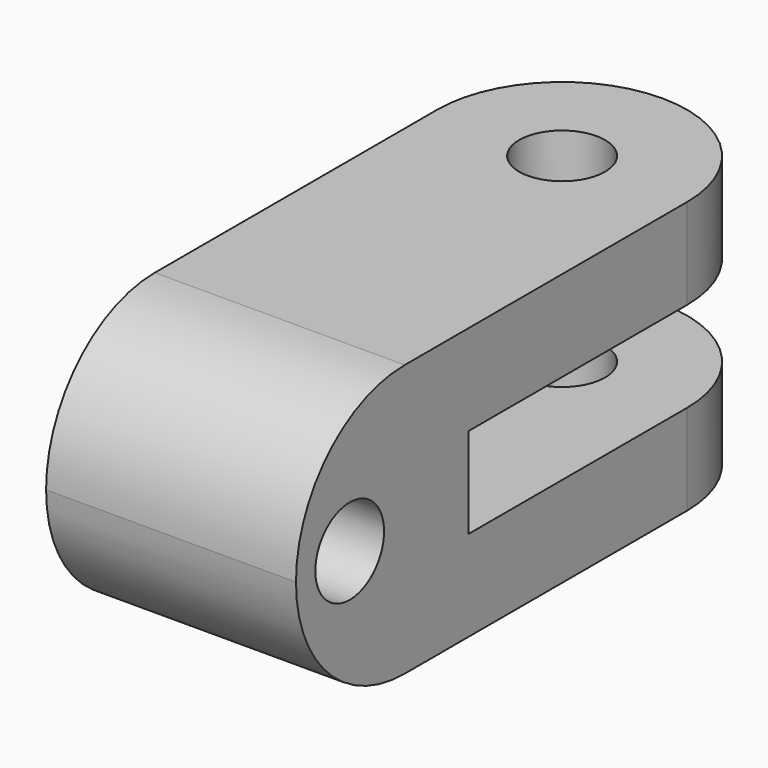
from build123d import *

# Parameters (mm, degrees)
F0_W     = 79.502
F0_H     = 44.196
F1_DEPTH = 40.64
F3_T     = -14.732
F4_D     = 13.97
F6_W     = 20.32
F6_H     = 44.196
F7_DEPTH = 40.64
F8_D     = 13.97
F9_R     = 22.09799
F10_R    = 20.31999


# Not quite as in the source:
# - a fillet or chamfer is up to 0.001 mm smaller than in the source, because OpenCascade refuses the exact size


with BuildPart() as f1:
    # F0 (on Right) → F1 (new body)
    with BuildSketch(Plane.YZ):
        with Locations((39.751, 22.098)):
            Rectangle(F0_W, F0_H)
    extrude(amount=F1_DEPTH)

    # F3
    f3_openings = [f1.faces().sort_by_distance(p)[0] for p in [
        (40.64, 39.751, 22.098),
        (20.32, 79.502, 22.098),
        (0, 39.751, 22.098),
    ]]
    offset(amount=F3_T, openings=f3_openings)

    # F4 (through all)
    with Locations(Plane.XY.offset(44.196)):
        with Locations((20.32, 59.182)):
            Hole(F4_D / 2)

    # F6 (on face) → F7 (join)
    with BuildSketch(Plane(origin=(0, 0, 0), x_dir=(0, -1, 0), z_dir=(-1, 0, 0))):
        with Locations((10.16, 22.098)):
            Rectangle(F6_W, F6_H)
    extrude(amount=-F7_DEPTH)

    # F8 (through all)
    with Locations(Plane.YZ.offset(40.64)):
        with Locations((-9.398, 22.098)):
            Hole(F8_D / 2)

    # F9 (radius 22.098 in the source; OpenCascade refuses exactly that, so slightly less here)
    f9_edges = [f1.edges().sort_by_distance(p)[0] for p in [
        (20.32, -20.32, 44.196),
        (20.32, -20.32, 0),
    ]]
    fillet(f9_edges, radius=F9_R)

    # F10 (radius 20.32 in the source; OpenCascade refuses exactly that, so slightly less here)
    f10_edges = [f1.edges().sort_by_distance(p)[0] for p in [
        (0, 79.502, 36.83),
        (0, 79.502, 7.366),
        (40.64, 79.502, 7.366),
        (40.64, 79.502, 36.83),
    ]]
    fillet(f10_edges, radius=F10_R)


solid = f1.part
